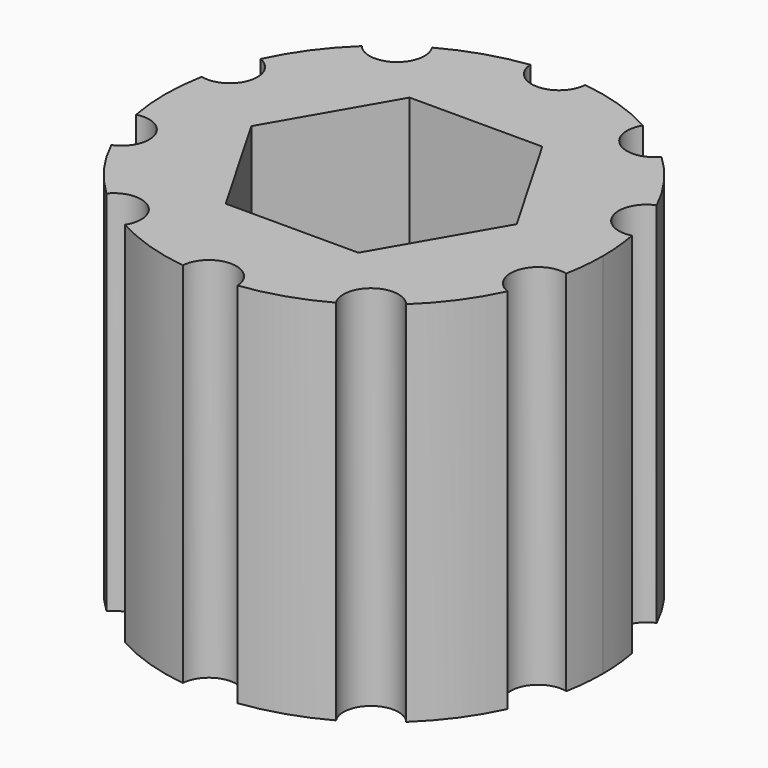
from build123d import *

# Parameters (mm, degrees)
F1_DEPTH = 16
F2_R     = 3
F3_DEPTH = 16.001
F4_R     = 3
F5_DEPTH = 6


with BuildPart() as f1:
    # F0 (on Top) → F1 (new body)
    with BuildSketch(Plane.XY):
        with BuildLine():
            ThreePointArc((9.3561974046, -1.7852717232), (9.4827054494, -0.8966171761), (9.525, 0))
            ThreePointArc((9.525, 0), (9.4827054494, 0.8966171761), (9.3561974046, 1.7852717232))
            ThreePointArc((9.3561974046, 1.7852717232), (7.9216471704, 2.5738991923), (8.6186790933, 4.0551196883))
            ThreePointArc((8.6186790933, 4.0551196883), (7.7058868714, 5.5986545281), (6.5199663128, 6.9437500156))
            ThreePointArc((6.5199663128, 6.9437500156), (4.8958471982, 6.738555569), (4.5891183065, 8.3465932074))
            ThreePointArc((4.5891183065, 8.3465932074), (2.9433868714, 9.0588133177), (1.193329695, 9.4499518115))
            ThreePointArc((1.193329695, 9.4499518115), (0, 8.3293127534), (-1.193329695, 9.4499518115))
            ThreePointArc((-1.193329695, 9.4499518115), (-2.9433868714, 9.0588133177), (-4.5891183065, 8.3465932074))
            ThreePointArc((-4.5891183065, 8.3465932074), (-4.4504477573, 8.039487236), (-4.4029672815, 7.7058868714))
            ThreePointArc((-4.4029672815, 7.7058868714), (-5.1936438859, 6.5808827064), (-6.5199663128, 6.9437500156))
            ThreePointArc((-6.5199663128, 6.9437500156), (-7.7058868714, 5.5986545281), (-8.6186790933, 4.0551196883))
            ThreePointArc((-8.6186790933, 4.0551196883), (-8.0698919683, 3.6154750772), (-7.8631260711, 2.9433868714))
            ThreePointArc((-7.8631260711, 2.9433868714), (-8.3259799016, 1.9985995007), (-9.3561974046, 1.7852717232))
            ThreePointArc((-9.3561974046, 1.7852717232), (-9.525, 0), (-9.3561974046, -1.7852717232))
            ThreePointArc((-9.3561974046, -1.7852717232), (-8.3259799016, -1.9985995007), (-7.8631260711, -2.9433868714))
            ThreePointArc((-7.8631260711, -2.9433868714), (-8.0698919683, -3.6154750772), (-8.6186790933, -4.0551196883))
            ThreePointArc((-8.6186790933, -4.0551196883), (-7.7058868714, -5.5986545281), (-6.5199663128, -6.9437500156))
            ThreePointArc((-6.5199663128, -6.9437500156), (-5.1936438859, -6.5808827064), (-4.4029672815, -7.7058868714))
            ThreePointArc((-4.4029672815, -7.7058868714), (-4.4504477573, -8.039487236), (-4.5891183065, -8.3465932074))
            ThreePointArc((-4.5891183065, -8.3465932074), (-2.9433868714, -9.0588133177), (-1.193329695, -9.4499518115))
            ThreePointArc((-1.193329695, -9.4499518115), (0, -8.3293127534), (1.193329695, -9.4499518115))
            ThreePointArc((1.193329695, -9.4499518115), (2.9433868714, -9.0588133177), (4.5891183065, -8.3465932074))
            ThreePointArc((4.5891183065, -8.3465932074), (4.8958471982, -6.738555569), (6.5199663128, -6.9437500156))
            ThreePointArc((6.5199663128, -6.9437500156), (7.7058868714, -5.5986545281), (8.6186790933, -4.0551196883))
            ThreePointArc((8.6186790933, -4.0551196883), (7.9216471704, -2.5738991923), (9.3561974046, -1.7852717232))
        make_face()
    extrude(amount=F1_DEPTH)

    # F2 (on face) → F3 (cut, through all)
    with BuildSketch(Plane.XY.offset(16)):
        Circle(F2_R)
    extrude(amount=-F3_DEPTH, mode=Mode.SUBTRACT)

    # F4 (on face) → F5 (cut)
    with BuildSketch(Plane.XY.offset(16)):
        Polygon((2.8867513459, -5), (5.7735026919, 0), (2.8867513459, 5), (-2.8867513459, 5), (-5.7735026919, 0), (-2.8867513459, -5), align=None)
        Circle(F4_R, mode=Mode.SUBTRACT)
    extrude(amount=-F5_DEPTH, mode=Mode.SUBTRACT)


solid = f1.part
